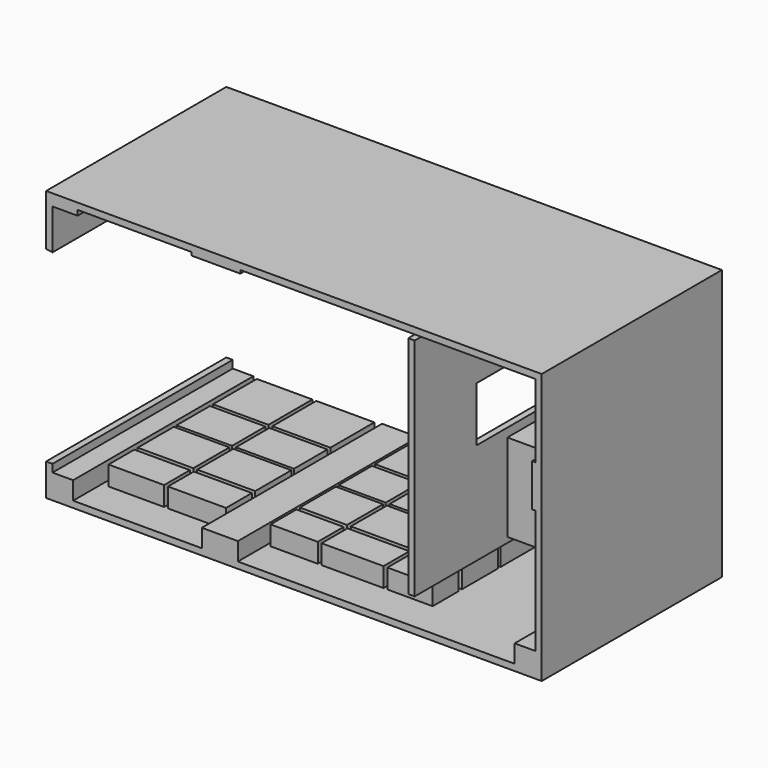
from build123d import *

# Parameters (mm, degrees)
F5_DEPTH  = 88.9
F3_W      = 2.54
F3_H      = 88.9
F1_W      = 139.7
F1_H      = 15.24
F8_DEPTH  = 25.4
F7_W      = 5.08
F7_H      = 21.59
F9_DEPTH  = 58.42
F2_W      = 20.32
F2_H      = 34.544
F10_DEPTH = 43.18
F11_W     = 21.9367220569
F11_H     = 12.7427842925
F11_H_2   = 17.8008489311
F11_W_2   = 22.9115727548
F11_H_3   = 16.5028721094
F11_H_4   = 21.655281503
F11_W_3   = 18.6136638447
F11_W_4   = 24.4355718235
F11_W_5   = 17.8599643318
F12_DEPTH = 7.62


# Not quite as in the source:
# - a feature of the source that left no trace in its solid (it failed there, or was rolled back) is left out
# - a feature names something its author has since deleted; it is built from what else it names


with BuildPart() as f5:
    # F0 (on Front) → F5 (new body)
    with BuildSketch(Plane.XZ):
        Polygon((-54.2084437874, 77.8652965117), (-54.2084437874, 79.8972965117), (-9.2940292287, 79.8972965117), (-9.2940292287, 78.6272965117), (10.0099707713, 78.6272965117), (10.0099707713, 79.8972965117), (126.3855562126, 79.8972965117), (126.3855562126, 50.9412965117), (125.1155562126, 50.9412965117), (125.1155562126, 34.1772965117), (126.3855562126, 34.1772965117), (126.3855562126, -14.5907034883), (118.2575562126, -14.5907034883), (118.2575562126, -21.7027034883), (9.0375562126, -21.7027034883), (9.0375562126, -14.5907034883), (-5.1864437874, -14.5907034883), (-5.1864437874, -21.7027034883), (-55.9864437874, -21.7027034883), (-55.9864437874, -14.5907034883), (-64.1144437874, -14.5907034883), (-64.1144437874, -11.5427034883), (-66.6544437874, -11.5427034883), (-66.6544437874, -24.2427034883), (128.9255562126, -24.2427034883), (128.9255562126, -21.7027034883), (128.9255562126, 82.4372965117), (-66.6544437874, 82.4372965117), (-66.6544437874, 62.2772533174), (-64.1144437874, 61.9093436475), (-64.1144437874, 77.8652965117), align=None)
    extrude(amount=F5_DEPTH)

    # F11 (on face) → F12 (join)
    with BuildSketch(Plane.XY.offset(-21.7027034883)):
        with Locations((-42.4272827589, -68.3046078538)):
            Rectangle(F11_W, F11_H)
        with Locations((-42.4272827589, -51.3639580458)):
            Rectangle(F11_W, F11_H_2)
        with Locations((-18.4791353531, -51.3639580458)):
            Rectangle(F11_W_2, F11_H_2)
        with Locations((-18.4791353531, -68.3046078538)):
            Rectangle(F11_W_2, F11_H)
        with Locations((-42.4272827589, -32.9141207039)):
            Rectangle(F11_W, F11_H_3)
        with Locations((-18.4791353531, -32.9141207039)):
            Rectangle(F11_W_2, F11_H_3)
        with Locations((-18.4791353531, -12.3516407515)):
            Rectangle(F11_W_2, F11_H_4)
        with Locations((-42.4272827589, -12.3516407515)):
            Rectangle(F11_W, F11_H_4)
        with Locations((19.868388135, -32.9141207039)):
            Rectangle(F11_W_3, F11_H_3)
        with Locations((19.868388135, -51.3639580458)):
            Rectangle(F11_W_3, F11_H_2)
        with Locations((19.868388135, -68.3046078538)):
            Rectangle(F11_W_3, F11_H)
        with Locations((42.9170059691, -68.3046078538)):
            Rectangle(F11_W_4, F11_H)
        with Locations((65.5887740467, -68.3046078538)):
            Rectangle(F11_W_5, F11_H)
        with Locations((65.5887740467, -51.3639580458)):
            Rectangle(F11_W_5, F11_H_2)
        with Locations((42.9170059691, -51.3639580458)):
            Rectangle(F11_W_4, F11_H_2)
        with Locations((42.9170059691, -32.9141207039)):
            Rectangle(F11_W_4, F11_H_3)
        with Locations((65.5887740467, -32.9141207039)):
            Rectangle(F11_W_5, F11_H_3)
        with Locations((65.5887740467, -12.3516407515)):
            Rectangle(F11_W_5, F11_H_4)
        with Locations((42.9170059691, -12.3516407515)):
            Rectangle(F11_W_4, F11_H_4)
        with Locations((19.868388135, -12.3516407515)):
            Rectangle(F11_W_3, F11_H_4)
    extrude(amount=F12_DEPTH)


with BuildPart() as f5b:
    # F3 (on Front) → F5, piece 2 (new body)
    with BuildSketch(Plane.XZ):
        with Locations((77.5370186973, 33.3226016507)):
            Rectangle(F3_W, F3_H)
    extrude(amount=F5_DEPTH)

    # F7 (on Front) → F9 (cut)
    with BuildSketch(Plane.XZ):
        with Locations((77.5194165921, 39.7443948221)):
            Rectangle(F7_W, F7_H)
    extrude(amount=F9_DEPTH, mode=Mode.SUBTRACT)

    # F2 (on Front) → F10 (join)
    with BuildSketch(Plane.XZ):
        with Locations((84.8901355004, 8.2332931607)):
            Rectangle(F2_W, F2_H)
    extrude(amount=F10_DEPTH)


with BuildPart() as f8:
    # F1 (on Front) → F8 (new body)
    with BuildSketch(Plane.XZ):
        with Locations((6.3137017131, 69.6807100427)):
            Rectangle(F1_W, F1_H)
    extrude(amount=F8_DEPTH)


solid = Compound([f5.part, f5b.part, f8.part])
